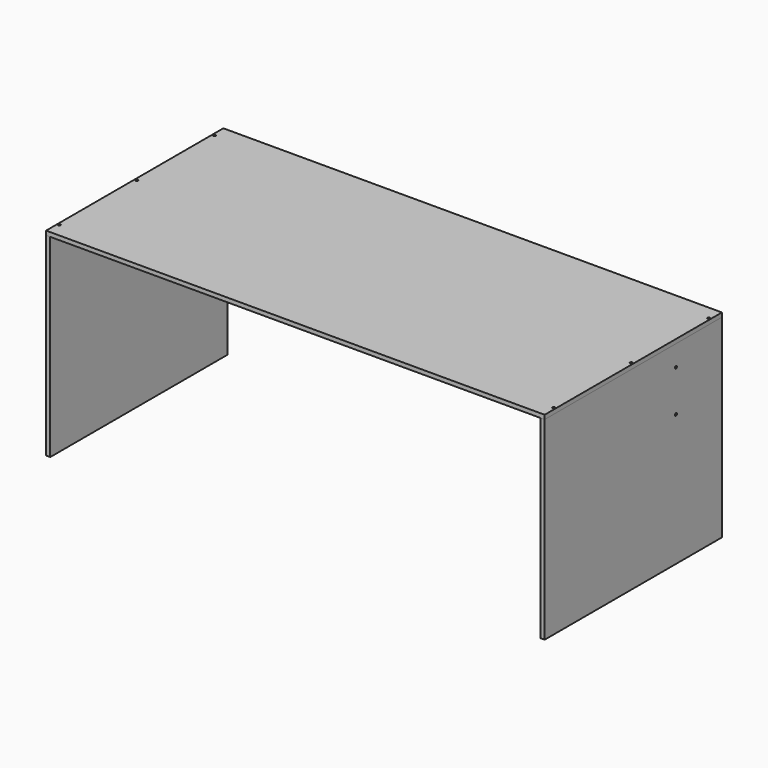
from build123d import *

# Parameters (mm, degrees)
F1_DEPTH          = 800
F0_W              = 15
F0_H              = 700
F2_DEPTH          = 800
F3_W              = 1770
F3_H              = 15
F4_DEPTH          = 300
F6_D              = 4
F6_DEPTH          = 20
F6_CSINK_D        = 8.96
F6_CSINK_ANGLE    = 90
F6_TIP            = 1.2017212381
F6_2_D            = 4
F6_2_DEPTH        = 20
F6_2_CSINK_D      = 8.96
F6_2_CSINK_ANGLE  = 90
F6_2_TIP          = 1.2017212381
F6_3_D            = 4
F6_3_DEPTH        = 20
F6_3_CSINK_D      = 8.96
F6_3_CSINK_ANGLE  = 90
F6_3_TIP          = 1.2017212381
F8_D              = 4
F8_DEPTH          = 40
F8_CSINK_D        = 8.96
F8_CSINK_ANGLE    = 90
F8_TIP            = 1.2017212381
F8_2_D            = 4
F8_2_DEPTH        = 40
F8_2_CSINK_D      = 8.96
F8_2_CSINK_ANGLE  = 90
F8_2_TIP          = 1.2017212381
F10_D             = 4
F10_DEPTH         = 40
F10_CSINK_D       = 8.96
F10_CSINK_ANGLE   = 90
F10_TIP           = 1.2017212381
F10_2_D           = 4
F10_2_DEPTH       = 40
F10_2_CSINK_D     = 8.96
F10_2_CSINK_ANGLE = 90
F10_2_TIP         = 1.2017212381
F12_D             = 3
F12_DEPTH         = 1
F12_TIP           = 0.9012909285
F12_2_D           = 3
F12_2_DEPTH       = 1
F12_2_TIP         = 0.9012909285


# Not quite as in the source:
# - a feature names something its author has since deleted; it is built from what else it names


with BuildPart() as f1:
    # F0 (on Front) → F1 (new body)
    with BuildSketch(Plane.XZ):
        Polygon((0, 15), (0, 0), (15, 0), (1785, 0), (1800, 0), (1800, 15), align=None)
    extrude(amount=-F1_DEPTH)

    # F6
    with Locations(Plane.XY.offset(15)):
        with Locations((7.5, 750), (7.5, 400), (7.5, 50), (1792.5, 750), (1792.5, 400), (1792.5, 50)):
            CounterSinkHole(F6_D / 2, F6_CSINK_D / 2, depth=F6_DEPTH, counter_sink_angle=F6_CSINK_ANGLE)
            with Locations((0, 0, -(F6_DEPTH + F6_TIP / 2))):  # 118° drill point
                Cone(0, F6_D / 2, F6_TIP, mode=Mode.SUBTRACT)


with BuildPart() as f2:
    # F0 (on Front) → F2 (new body)
    with BuildSketch(Plane.XZ):
        with Locations((7.5, -350)):
            Rectangle(F0_W, F0_H)
    extrude(amount=-F2_DEPTH)

    # F6#2
    with Locations(Plane.XY.offset(15)):
        with Locations((7.5, 750), (7.5, 400), (7.5, 50), (1792.5, 750), (1792.5, 400), (1792.5, 50)):
            CounterSinkHole(F6_2_D / 2, F6_2_CSINK_D / 2, depth=F6_2_DEPTH, counter_sink_angle=F6_2_CSINK_ANGLE)
            with Locations((0, 0, -(F6_2_DEPTH + F6_2_TIP / 2))):  # 118° drill point
                Cone(0, F6_2_D / 2, F6_2_TIP, mode=Mode.SUBTRACT)

    # F8
    with Locations(Plane(origin=(0, 0, 0), x_dir=(0, -1, 0), z_dir=(-1, 0, 0))):
        with Locations((-592.5, -75), (-592.5, -225)):
            CounterSinkHole(F8_D / 2, F8_CSINK_D / 2, depth=F8_DEPTH, counter_sink_angle=F8_CSINK_ANGLE)
            with Locations((0, 0, -(F8_DEPTH + F8_TIP / 2))):  # 118° drill point
                Cone(0, F8_D / 2, F8_TIP, mode=Mode.SUBTRACT)

    # F12
    with Locations(Plane(origin=(0, 0, -700), x_dir=(1, 0, 0), z_dir=(0, 0, -1))):
        with Locations((1792.5, -30), (1792.5, -770), (7.5, -30), (7.5, -770)):
            Hole(F12_D / 2, depth=F12_DEPTH)
            with Locations((0, 0, -(F12_DEPTH + F12_TIP / 2))):  # 118° drill point
                Cone(0, F12_D / 2, F12_TIP, mode=Mode.SUBTRACT)


with BuildPart() as f2b:
    # F0 (on Front) → F2, piece 2 (new body)
    with BuildSketch(Plane.XZ):
        with Locations((1792.5, -350)):
            Rectangle(F0_W, F0_H)
    extrude(amount=-F2_DEPTH)

    # F6#3
    with Locations(Plane.XY.offset(15)):
        with Locations((7.5, 750), (7.5, 400), (7.5, 50), (1792.5, 750), (1792.5, 400), (1792.5, 50)):
            CounterSinkHole(F6_3_D / 2, F6_3_CSINK_D / 2, depth=F6_3_DEPTH, counter_sink_angle=F6_3_CSINK_ANGLE)
            with Locations((0, 0, -(F6_3_DEPTH + F6_3_TIP / 2))):  # 118° drill point
                Cone(0, F6_3_D / 2, F6_3_TIP, mode=Mode.SUBTRACT)

    # F10
    with Locations(Plane.YZ.offset(1800)):
        with Locations((592.5, -75), (592.5, -225)):
            CounterSinkHole(F10_D / 2, F10_CSINK_D / 2, depth=F10_DEPTH, counter_sink_angle=F10_CSINK_ANGLE)
            with Locations((0, 0, -(F10_DEPTH + F10_TIP / 2))):  # 118° drill point
                Cone(0, F10_D / 2, F10_TIP, mode=Mode.SUBTRACT)

    # F12#2
    with Locations(Plane(origin=(0, 0, -700), x_dir=(1, 0, 0), z_dir=(0, 0, -1))):
        with Locations((1792.5, -30), (1792.5, -770), (7.5, -30), (7.5, -770)):
            Hole(F12_2_D / 2, depth=F12_2_DEPTH)
            with Locations((0, 0, -(F12_2_DEPTH + F12_2_TIP / 2))):  # 118° drill point
                Cone(0, F12_2_D / 2, F12_2_TIP, mode=Mode.SUBTRACT)


with BuildPart() as f4:
    # F3 (on face) → F4 (new body)
    with BuildSketch(Plane(origin=(0, 0, 0), x_dir=(1, 0, 0), z_dir=(0, 0, -1))):
        with Locations((900, -592.5)):
            Rectangle(F3_W, F3_H)
    extrude(amount=F4_DEPTH)

    # F8#2
    with Locations(Plane(origin=(0, 0, 0), x_dir=(0, -1, 0), z_dir=(-1, 0, 0))):
        with Locations((-592.5, -75), (-592.5, -225)):
            CounterSinkHole(F8_2_D / 2, F8_2_CSINK_D / 2, depth=F8_2_DEPTH, counter_sink_angle=F8_2_CSINK_ANGLE)
            with Locations((0, 0, -(F8_2_DEPTH + F8_2_TIP / 2))):  # 118° drill point
                Cone(0, F8_2_D / 2, F8_2_TIP, mode=Mode.SUBTRACT)

    # F10#2
    with Locations(Plane.YZ.offset(1800)):
        with Locations((592.5, -75), (592.5, -225)):
            CounterSinkHole(F10_2_D / 2, F10_2_CSINK_D / 2, depth=F10_2_DEPTH, counter_sink_angle=F10_2_CSINK_ANGLE)
            with Locations((0, 0, -(F10_2_DEPTH + F10_2_TIP / 2))):  # 118° drill point
                Cone(0, F10_2_D / 2, F10_2_TIP, mode=Mode.SUBTRACT)


solid = Compound([f1.part, f2.part, f2b.part, f4.part])
